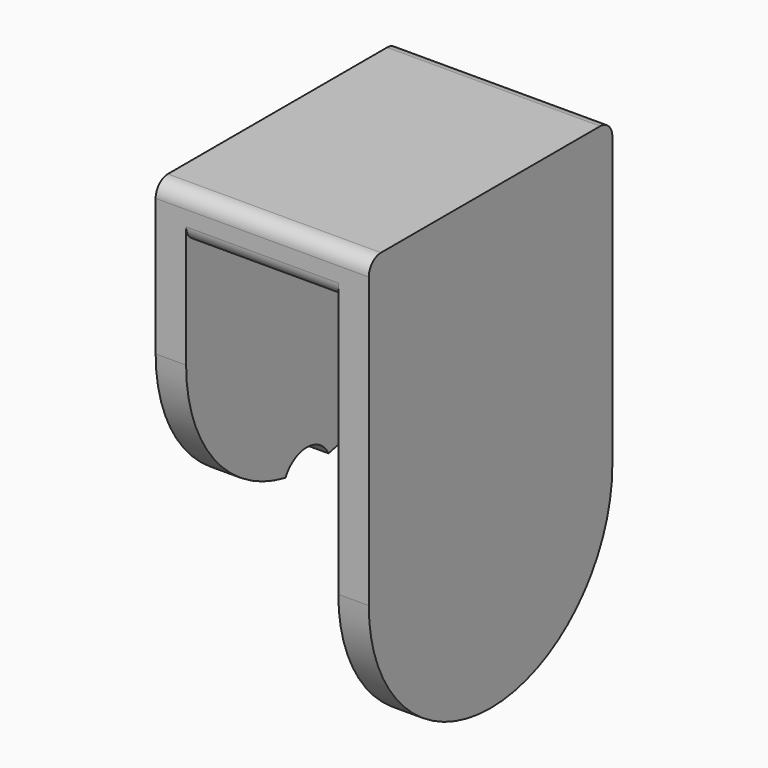
from build123d import *

# Parameters (mm, degrees)
F0_W     = 10
F0_H     = 3
F1_DEPTH = 20
F2_R     = 9.99999
F4_D     = 4
F4_DEPTH = 12.1423804591
F5_R     = 1


# Not quite as in the source:
# - a fillet or chamfer is up to 0.001 mm smaller than in the source, because OpenCascade refuses the exact size


with BuildPart() as f1:
    # F0 (on Front) → F1 (new body)
    with BuildSketch(Plane.XZ):
        with Locations((-5.1413804591, 1.5)):
            Rectangle(F0_W, F0_H)
        Polygon((-10.1413804591, 0), (-10.1413804591, 3), (-12.1413804591, 3), (-12.1413804591, -17), (-10.1413804591, -17), align=None)
        Polygon((1.8586195409, 3), (-0.1413804591, 3), (-0.1413804591, 0), (-0.1413804591, -27), (1.8586195409, -27), align=None)
    extrude(amount=F1_DEPTH)

    # F2 (radius 10 in the source; OpenCascade refuses exactly that, so slightly less here)
    f2_edges = [f1.edges().sort_by_distance(p)[0] for p in [
        (-11.14138, 0, -17),
        (-11.14138, -20, -17),
        (0.85862, -20, -27),
        (0.85862, 0, -27),
    ]]
    fillet(f2_edges, radius=F2_R)

    # F4 (through all, one way)
    with BuildSketch(Plane.YZ):
        with Locations((-10.0830290467, -17.7759565413)):
            Circle(F4_D / 2)
    extrude(amount=-F4_DEPTH, mode=Mode.SUBTRACT)

    # F5
    f5_edges = [f1.edges().sort_by_distance(p)[0] for p in [
        (-5.14138, 0, 0),
        (-5.14138, -20, 0),
        (-5.14138, -20, 3),
        (-5.14138, 0, 3),
    ]]
    fillet(f5_edges, radius=F5_R)


solid = f1.part
